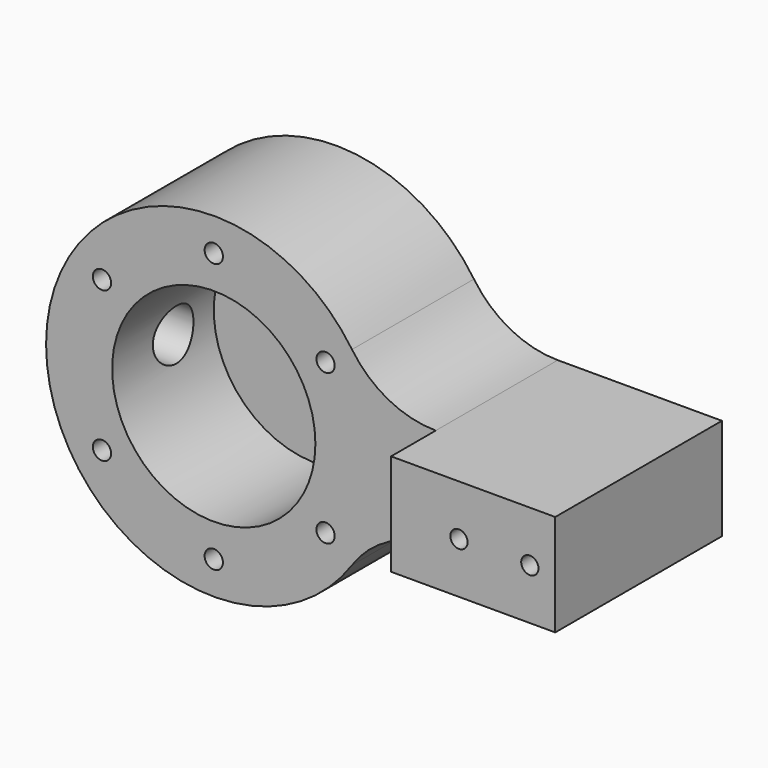
from build123d import *

# Parameters (mm, degrees)
F0_R           = 33
F1_DEPTH       = 5
F2_R           = 33
F2_R_2         = 20
F3_DEPTH       = 25
F4_R           = 1.8
F5_DEPTH       = 30.001
F7_W           = 20
F7_H           = 20
F8_DEPTH       = 52
F9_W           = 52
F9_H           = 20
F12_DEPTH      = 10
F11_R          = 5
F13_DEPTH      = 12.001
F13_DEPTH_BACK = 10
F14_R          = 20
F15_W          = 20
F15_H          = 20
F16_DEPTH      = 11
F17_R          = 1.7
F18_DEPTH      = 41.0010001
F19_W          = 17.3078954501
F19_H          = 20
F20_DEPTH      = 11
F21_R          = 1.7
F22_DEPTH      = 41.0010001
F23_W          = 5
F23_H          = 20
F24_DEPTH      = 41.0010001


# Not quite as in the source:
# - a feature names something its author has since deleted; it is built from what else it names


with BuildPart() as f1:
    # F0 (on Front) → F1 (new body)
    with BuildSketch(Plane.XZ):
        Circle(F0_R)
    extrude(amount=F1_DEPTH)

    # F2 (on face) → F3 (join)
    with BuildSketch(Plane.XZ.offset(5)):
        Circle(F2_R)
        Circle(F2_R_2, mode=Mode.SUBTRACT)
    extrude(amount=F3_DEPTH)

    # F4 (on face) → F5 (cut, through all)
    with BuildSketch(Plane.XZ.offset(30)):
        with Locations((0, 26.5)):
            Circle(F4_R)
        with Locations((22, 14.7732867027)):
            Circle(F4_R)
        with Locations((-22, 14.7732867027)):
            Circle(F4_R)
        with Locations((0, -26.5)):
            Circle(F4_R)
        with Locations((-22, -14.7732867027)):
            Circle(F4_R)
        with Locations((22, -14.7732867027)):
            Circle(F4_R)
    extrude(amount=-F5_DEPTH, mode=Mode.SUBTRACT)

    # F7 (on offset) → F8 (join)
    with BuildSketch(Plane.YZ.offset(29)):
        with Locations((-10, 0)):
            Rectangle(F7_W, F7_H)
    extrude(amount=F8_DEPTH)

    # F9 (on face) → F12 (join)
    with BuildSketch(Plane.XZ.offset(20)):
        with Locations((55, 0)):
            Rectangle(F9_W, F9_H)
    extrude(amount=F12_DEPTH)

    # F11 (on offset) → F13 (cut, two sides)
    with BuildSketch(Plane.YZ.offset(-21)) as f13_sk:
        with Locations((-15, 0)):
            Circle(F11_R)
    extrude(amount=-F13_DEPTH, mode=Mode.SUBTRACT)
    extrude(f13_sk.sketch, amount=F13_DEPTH_BACK, mode=Mode.SUBTRACT)

    # F14
    f14_edges = [f1.edges().sort_by_distance(p)[0] for p in [
        (31.44837, -15, -10),
        (31.44837, -15, 10),
    ]]
    fillet(f14_edges, radius=F14_R)

    # F15 (on face) → F16 (join)
    with BuildSketch(Plane.XZ.offset(30)):
        with Locations((71, 0)):
            Rectangle(F15_W, F15_H)
    extrude(amount=F16_DEPTH)

    # F17 (on face) → F18 (cut, through all)
    with BuildSketch(Plane.XZ.offset(41)):
        with Locations((71, 0)):
            Circle(F17_R)
    extrude(amount=-F18_DEPTH, mode=Mode.SUBTRACT)

    # F19 (on face) → F20 (join)
    with BuildSketch(Plane.XZ.offset(30)):
        with Locations((52.346052275, 0)):
            Rectangle(F19_W, F19_H)
    extrude(amount=F20_DEPTH)

    # F21 (on face) → F22 (cut, through all)
    with BuildSketch(Plane.XZ.offset(41)):
        with Locations((57.05, 0)):
            Circle(F21_R)
    extrude(amount=-F22_DEPTH, mode=Mode.SUBTRACT)

    # F23 (on face) → F24 (cut, through all)
    with BuildSketch(Plane.XZ.offset(41)):
        with Locations((78.5, 0)):
            Rectangle(F23_W, F23_H)
    extrude(amount=-F24_DEPTH, mode=Mode.SUBTRACT)


solid = f1.part
